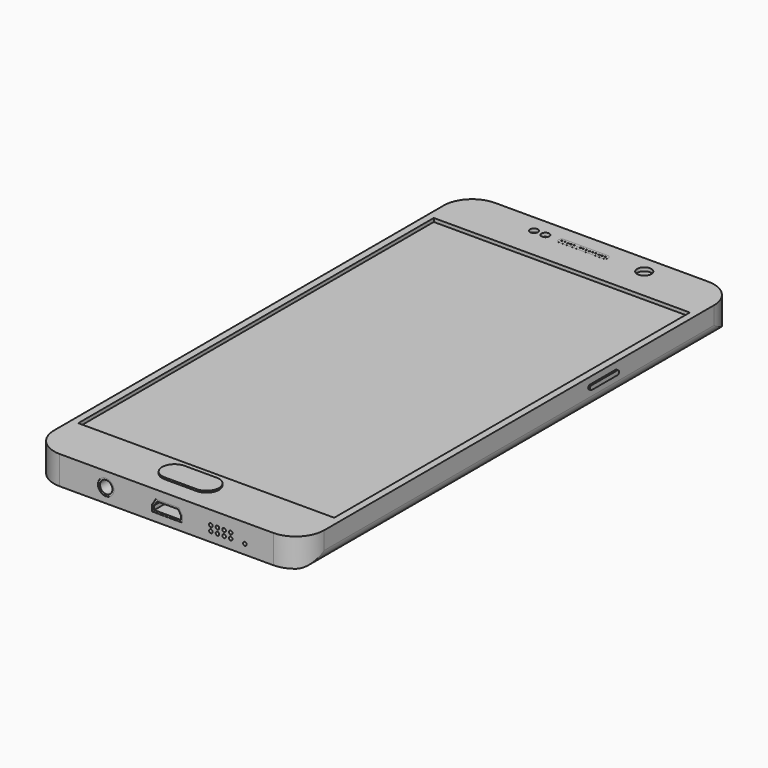
from build123d import *

# Parameters (mm, degrees)
F0_W         = 76
F0_H         = 153
F1_DEPTH     = 8
F2_W         = 72
F2_H         = 125
F3_DEPTH     = 1
F5_DEPTH     = 0.5
F6_R         = 1.1
F6_R_2       = 2
F7_DEPTH     = 1
F9_DEPTH     = 0.01
F10_R        = 0.2
F11_DEPTH    = 0.1
F13_DEPTH    = 0.5
F15_DEPTH    = 0.5
F16_R        = 2.25
F17_DEPTH    = 0.1
F18_R        = 1.75
F19_DEPTH    = 10
F21_DEPTH    = 0.1
F23_DEPTH    = 5
F24_R        = 0.5
F25_DEPTH    = 10
F27_DEPTH    = 2
F28_SIZE     = 1.8
F29_SIZE     = 0.2
F31_DEPTH    = 2
F32_R        = 1.5
F33_DEPTH    = 2
F35_DEPTH    = 1
F36_T1_DEPTH = 48.0048284771
F37_T1_DEPTH = 152.1580802856


# Not quite as in the source:
# - a fillet or chamfer that OpenCascade refuses, or shapes differently, is made with other operations: its cross-section is extruded or revolved along the edge and cut away or added
# - ends of sketch curves that miss each other by under 0.0002 mm in the source are joined


with BuildPart() as f1:
    # F0 (on Top) → F1 (new body)
    with BuildSketch(Plane.XY):
        Rectangle(F0_W, F0_H)
    extrude(amount=F1_DEPTH)

    # F2 (on face) → F3 (cut)
    with BuildSketch(Plane.XY.offset(8)):
        Rectangle(F2_W, F2_H)
    extrude(amount=-F3_DEPTH, mode=Mode.SUBTRACT)

    # F4 (on face) → F5 (join)
    with BuildSketch(Plane.XY.offset(8)):
        with BuildLine():
            Line((4.5, -64.5), (-4.5, -64.5))
            ThreePointArc((-4.5, -64.5), (-8, -68), (-4.5, -71.5))
            Line((-4.5, -71.5), (4.5, -71.5))
            ThreePointArc((4.5, -71.5), (8, -68), (4.5, -64.5))
        make_face()
    extrude(amount=F5_DEPTH)

    # F6 (on face) → F7 (cut)
    with BuildSketch(Plane.XY.offset(8)):
        with Locations((-15, 71.5)):
            Circle(F6_R)
        with Locations((-11.8, 71.5)):
            Circle(F6_R)
        with Locations((16, 71.5)):
            Circle(F6_R_2)
    extrude(amount=-F7_DEPTH, mode=Mode.SUBTRACT)

    # F8 (on face) → F9 (join)
    with BuildSketch(Plane.XY.offset(8)):
        with BuildLine():
            Line((5, 72.4), (-7.2, 72.4))
            ThreePointArc((-7.2, 72.4), (-8.1, 71.5), (-7.2, 70.6))
            Line((-7.2, 70.6), (5, 70.6))
            ThreePointArc((5, 70.6), (5.9, 71.5), (5, 72.4))
        make_face()
    extrude(amount=F9_DEPTH)

    # F10 (on face) → F11 (cut)
    with BuildSketch(Plane.XY.offset(8.01)):
        with Locations((-1.1, 71.5)):
            Circle(F10_R)
        with Locations((-7.2, 71.5)):
            Circle(F10_R)
        with Locations((5, 71.5)):
            Circle(F10_R)
        with Locations((-6.33, 71.5)):
            Circle(F10_R)
        with Locations((-5.46, 71.5)):
            Circle(F10_R)
        with Locations((-4.59, 71.5)):
            Circle(F10_R)
        with Locations((-3.71, 71.5)):
            Circle(F10_R)
        with Locations((-2.84, 71.5)):
            Circle(F10_R)
        with Locations((-1.97, 71.5)):
            Circle(F10_R)
        with Locations((-0.23, 71.5)):
            Circle(F10_R)
        with Locations((0.64, 71.5)):
            Circle(F10_R)
        with Locations((1.51, 71.5)):
            Circle(F10_R)
        with Locations((2.39, 71.5)):
            Circle(F10_R)
        with Locations((3.26, 71.5)):
            Circle(F10_R)
        with Locations((4.13, 71.5)):
            Circle(F10_R)
    extrude(amount=-F11_DEPTH, mode=Mode.SUBTRACT)

    # F12 (on face) → F13 (join)
    with BuildSketch(Plane(origin=(-38, 0, 0), x_dir=(0, -1, 0), z_dir=(-1, 0, 0))):
        with BuildLine():
            Line((-43.9, 6.1), (-52.9, 6.1))
            ThreePointArc((-52.9, 6.1), (-53.5, 5.5), (-52.9, 4.9))
            Line((-52.9, 4.9), (-43.9, 4.9))
            ThreePointArc((-43.9, 4.9), (-43.3, 5.5), (-43.9, 6.1))
        make_face()
        with BuildLine():
            Line((-29.7, 6.1), (-38.7, 6.1))
            ThreePointArc((-38.7, 6.1), (-39.3, 5.5), (-38.7, 4.9))
            Line((-38.7, 4.9), (-29.7, 4.9))
            ThreePointArc((-29.7, 4.9), (-29.1, 5.5), (-29.7, 6.1))
        make_face()
    extrude(amount=F13_DEPTH)

    # F14 (on face) → F15 (join)
    with BuildSketch(Plane.YZ.offset(38)):
        with BuildLine():
            ThreePointArc((24.8999994173, 4.9), (25.324263486, 5.0757359313), (25.4999994173, 5.5))
            ThreePointArc((25.4999994173, 5.5), (25.324263486, 5.9242640687), (24.8999994173, 6.1))
            ThreePointArc((24.8999994173, 6.1), (24.2999994173, 5.5), (24.8999994173, 4.9))
        make_face()
        with BuildLine():
            ThreePointArc((24.8999994173, 6.1), (25.324263486, 5.9242640687), (25.4999994173, 5.5))
            ThreePointArc((25.4999994173, 5.5), (25.324263486, 5.0757359313), (24.8999994173, 4.9))
            Line((24.8999994173, 4.9), (33.8999994173, 4.9))
            ThreePointArc((33.8999994173, 4.9), (33.2999988346, 5.5), (33.8999994173, 6.1000005827))
            Line((33.8999994173, 6.1000005827), (24.8999994173, 6.1))
        make_face()
        with BuildLine():
            ThreePointArc((34.5, 5.5), (34.324263898, 5.9242644808), (33.8999994173, 6.1000005827))
            ThreePointArc((33.8999994173, 6.1000005827), (33.2999988346, 5.5), (33.8999994173, 4.8999994173))
            ThreePointArc((33.8999994173, 4.8999994173), (34.324263898, 5.0757355192), (34.5, 5.5))
        make_face()
    extrude(amount=F15_DEPTH)

    # F16 (on face) → F17 (cut)
    with BuildSketch(Plane.XZ.offset(76.5)):
        with Locations((-17, 4)):
            Circle(F16_R)
    extrude(amount=-F17_DEPTH, mode=Mode.SUBTRACT)

    # F18 (on face) → F19 (cut)
    with BuildSketch(Plane.XZ.offset(76.4)):
        with Locations((-17, 4)):
            Circle(F18_R)
    extrude(amount=-F19_DEPTH, mode=Mode.SUBTRACT)

    # F20 (on face) → F21 (cut)
    with BuildSketch(Plane.XZ.offset(76.5)):
        Polygon((3.5, 5.6), (0.25, 5.6), (-3, 5.6), (-4, 4), (-4, 2.2), (0.25, 2.2), (4.5, 2.2), (4.5, 4), align=None)
    extrude(amount=-F21_DEPTH, mode=Mode.SUBTRACT)

    # F22 (on face) → F23 (cut)
    with BuildSketch(Plane.XZ.offset(76.4)):
        Polygon((3.2228761792, 5.1), (0.25, 5.1), (-2.7228761792, 5.1), (-3.5, 3.8566018868), (-3.5, 2.7), (0.25, 2.7), (4, 2.7), (4, 3.8566018868), align=None)
    extrude(amount=-F23_DEPTH, mode=Mode.SUBTRACT)

    # F24 (on face) → F25 (cut)
    with BuildSketch(Plane.XZ.offset(76.5)):
        with Locations((12.5, 4.2)):
            Circle(F24_R)
        with Locations((14.36, 4.2)):
            Circle(F24_R)
        with Locations((16.22, 4.2)):
            Circle(F24_R)
        with Locations((18.08, 4.2)):
            Circle(F24_R)
        with Locations((18.08, 2.7)):
            Circle(F24_R)
        with Locations((16.22, 2.7)):
            Circle(F24_R)
        with Locations((14.36, 2.7)):
            Circle(F24_R)
        with Locations((12.5, 2.7)):
            Circle(F24_R)
        with Locations((22.08, 2.7)):
            Circle(F24_R)
    extrude(amount=-F25_DEPTH, mode=Mode.SUBTRACT)

    # F26 (on face) → F27 (join)
    with BuildSketch(Plane(origin=(0, 0, 0), x_dir=(1, 0, 0), z_dir=(0, 0, -1))):
        with BuildLine():
            Line((-2, -61.5), (4, -61.5))
            ThreePointArc((4, -61.5), (7.5355339059, -60.0355339059), (9, -56.5))
            Line((9, -56.5), (9, -50.5))
            ThreePointArc((9, -50.5), (7.5355339059, -46.9644660941), (4, -45.5))
            Line((4, -45.5), (-2, -45.5))
            ThreePointArc((-2, -45.5), (-5.5355339059, -46.9644660941), (-7, -50.5))
            Line((-7, -50.5), (-7, -56.5))
            ThreePointArc((-7, -56.5), (-5.5355339059, -60.0355339059), (-2, -61.5))
        make_face()
    extrude(amount=F27_DEPTH)

    # F28
    f28_edges = [f1.edges().sort_by_distance(p)[0] for p in [
        (9, 53.5, -2),
        (-7, 53.5, -2),
        (-5.535534, 46.964466, -2),
        (1, 45.5, -2),
        (7.535534, 46.964466, -2),
        (7.535534, 60.035534, -2),
        (1, 61.5, -2),
        (-5.535534, 60.035534, -2),
    ]]
    chamfer(f28_edges, length=F28_SIZE)

    # F29
    f29_edges = [f1.edges().sort_by_distance(p)[0] for p in [
        (6.262742, 58.762742, -2),
        (-5.2, 53.5, -2),
        (-4.262742, 48.237258, -2),
        (7.2, 53.5, -2),
        (6.262742, 48.237258, -2),
        (1, 59.7, -2),
        (1, 47.3, -2),
        (-4.262742, 58.762742, -2),
    ]]
    chamfer(f29_edges, length=F29_SIZE)

    # F30 (on face) → F31 (cut)
    with BuildSketch(Plane(origin=(0, 0, -2), x_dir=(1, 0, 0), z_dir=(0, 0, -1))):
        with BuildLine():
            Line((-4.8, -50.5), (-4.8, -56.5))
            ThreePointArc((-4.8, -56.5), (-3.9798989873, -58.4798989873), (-2, -59.3))
            Line((-2, -59.3), (4, -59.3))
            ThreePointArc((4, -59.3), (5.9798989873, -58.4798989873), (6.8, -56.5))
            Line((6.8, -56.5), (6.8, -50.5))
            ThreePointArc((6.8, -50.5), (5.9798989873, -48.5201010127), (4, -47.7))
            Line((4, -47.7), (-2, -47.7))
            ThreePointArc((-2, -47.7), (-3.9798989873, -48.5201010127), (-4.8, -50.5))
        make_face()
    extrude(amount=-F31_DEPTH, mode=Mode.SUBTRACT)

    # F32 (on face) → F33 (cut)
    with BuildSketch(Plane(origin=(0, 0, 0), x_dir=(1, 0, 0), z_dir=(0, 0, -1))):
        with Locations((1, -53.5)):
            Circle(F32_R)
    extrude(amount=-F33_DEPTH, mode=Mode.SUBTRACT)

    # F34 (on face) → F35 (cut)
    with BuildSketch(Plane(origin=(0, 0, 0), x_dir=(1, 0, 0), z_dir=(0, 0, -1))):
        with BuildLine():
            ThreePointArc((-17.5, -58), (-17.0606601718, -59.0606601718), (-16, -59.5))
            Line((-16, -59.5), (-14, -59.5))
            ThreePointArc((-14, -59.5), (-12.9393398282, -59.0606601718), (-12.5, -58))
            Line((-12.5, -58), (-12.5, -49))
            ThreePointArc((-12.5, -49), (-12.9393398282, -47.9393398282), (-14, -47.5))
            Line((-14, -47.5), (-16, -47.5))
            ThreePointArc((-16, -47.5), (-17.0606601718, -47.9393398282), (-17.5, -49))
            Line((-17.5, -49), (-17.5, -58))
        make_face()
    extrude(amount=-F35_DEPTH, mode=Mode.SUBTRACT)

    # F36: fillet of radius 8 on 4 edges, made by hand

    # F36_s2 → F36_t1 (cut)
    with BuildSketch(Plane.XY.offset(-20.0024142386)):
        with BuildLine():
            ThreePointArc((29.9990343146, 76.5004), (35.6568542495, 74.1568542495), (38.0004, 68.4990343146))
            Line((38.0004, 68.4990343146), (38.8005365685, 68.4990343146))
            ThreePointArc((38.8005365685, 68.4990343146), (38.8001365685, 72.4995171573), (38.8001365685, 76.5))
            Line((38.8001365685, 76.5), (38, 77.3001365685))
            ThreePointArc((38, 77.3001365685), (33.9995171573, 77.3001365685), (29.9990343146, 77.3005365685))
            Line((29.9990343146, 77.3005365685), (29.9990343146, 76.5004))
        make_face()
        with BuildLine():
            ThreePointArc((-29.9990343146, 76.5004), (-35.6568542495, 74.1568542495), (-38.0004, 68.4990343146))
            Line((-38.0004, 68.4990343146), (-38.8005365685, 68.4990343146))
            ThreePointArc((-38.8005365685, 68.4990343146), (-38.8001365685, 72.4995171573), (-38.8001365685, 76.5))
            Line((-38.8001365685, 76.5), (-38, 77.3001365685))
            ThreePointArc((-38, 77.3001365685), (-33.9995171573, 77.3001365685), (-29.9990343146, 77.3005365685))
            Line((-29.9990343146, 77.3005365685), (-29.9990343146, 76.5004))
        make_face()
        with BuildLine():
            ThreePointArc((-38.0004, -68.4990343146), (-35.6568542495, -74.1568542495), (-29.9990343146, -76.5004))
            Line((-29.9990343146, -76.5004), (-29.9990343146, -77.3005365685))
            ThreePointArc((-29.9990343146, -77.3005365685), (-33.9995171573, -77.3001365685), (-38, -77.3001365685))
            Line((-38, -77.3001365685), (-38.8001365685, -76.5))
            ThreePointArc((-38.8001365685, -76.5), (-38.8001365685, -72.4995171573), (-38.8005365685, -68.4990343146))
            Line((-38.8005365685, -68.4990343146), (-38.0004, -68.4990343146))
        make_face()
        with BuildLine():
            ThreePointArc((38.0004, -68.4990343146), (35.6568542495, -74.1568542495), (29.9990343146, -76.5004))
            Line((29.9990343146, -76.5004), (29.9990343146, -77.3005365685))
            ThreePointArc((29.9990343146, -77.3005365685), (33.9995171573, -77.3001365685), (38, -77.3001365685))
            Line((38, -77.3001365685), (38.8001365685, -76.5))
            ThreePointArc((38.8001365685, -76.5), (38.8001365685, -72.4995171573), (38.8005365685, -68.4990343146))
            Line((38.8005365685, -68.4990343146), (38.0004, -68.4990343146))
        make_face()
    extrude(amount=F36_T1_DEPTH, mode=Mode.SUBTRACT)

    # F37: fillet of radius 3 on 2 edges, made by hand

    # F37_s2 → F37_t1 (cut)
    with BuildSketch(Plane.XZ.offset(-76.0790401428)):
        with BuildLine():
            ThreePointArc((35, 0), (37.1213203436, 0.8786796564), (38, 3))
            Line((38, 3), (38, 0))
            Line((38, 0), (35, 0))
        make_face()
        with BuildLine():
            ThreePointArc((-35, 0), (-37.1213203436, 0.8786796564), (-38, 3))
            Line((-38, 3), (-38, 0))
            Line((-38, 0), (-35, 0))
        make_face()
    extrude(amount=F37_T1_DEPTH, mode=Mode.SUBTRACT)


solid = f1.part
